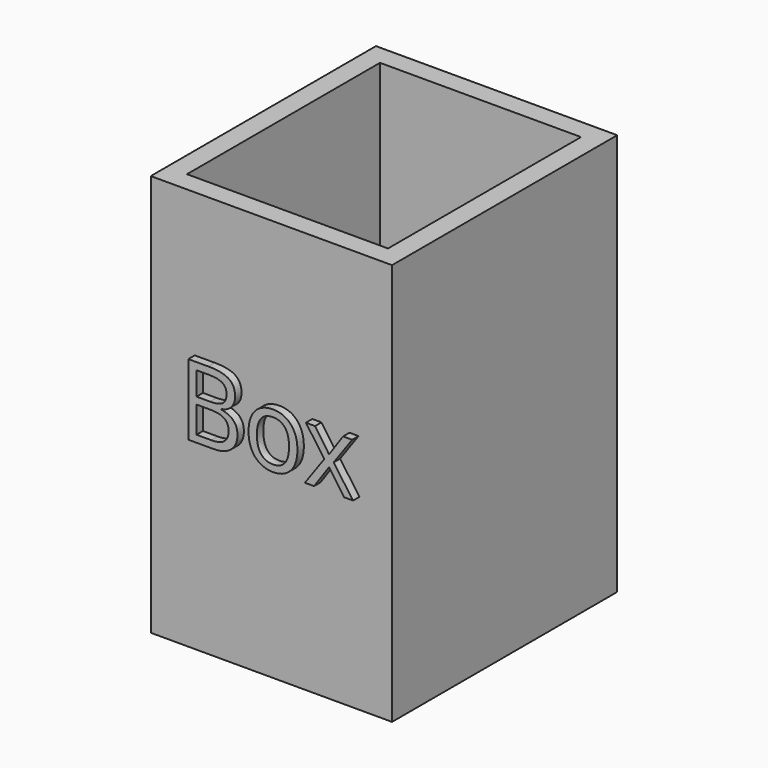
from build123d import *

# Parameters (mm, degrees)
F0_W         = 76.2
F0_H         = 127
F1_DEPTH     = 88.9
F2_T         = -6.35
F3_TEXT_SIZE = 31.4004596375
F4_DEPTH     = 2.54


# Not quite as in the source:
# - Text() gives the source's letters only with a copy of the font that has no kerning and outlines rounded to 1/6400 em; it was checked with that copy


with BuildPart() as f1:
    # F0 (on Front) → F1 (new body)
    with BuildSketch(Plane.XZ):
        Rectangle(F0_W, F0_H)
    extrude(amount=F1_DEPTH)

    # F2
    f2_openings = [f1.faces().sort_by_distance(p)[0] for p in [
        (0, -44.45, 63.5),
    ]]
    offset(amount=F2_T, openings=f2_openings)

    # F3 (on face) → F4 (join)
    with BuildSketch(Plane.XZ.offset(88.9)):
        with Locations((-27.3061655462, -4.257413093)):
            Text('Box', F3_TEXT_SIZE, font='Open Sans', text_align=(TextAlign.LEFT, TextAlign.BOTTOM))
    extrude(amount=F4_DEPTH)


solid = f1.part
